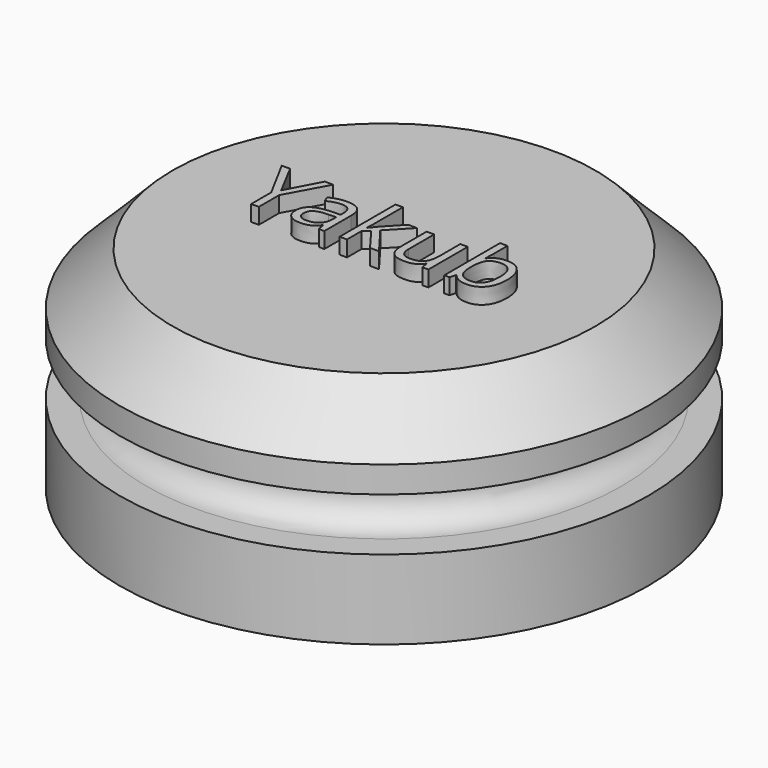
from build123d import *

# Parameters (mm, degrees)
F2_SIZE      = 1
F3_W         = 3.4
F3_H         = 1.1
F4_DEPTH     = 3
F5_R         = 0.49999
F6_TEXT_SIZE = 1.7380913584
F7_DEPTH     = 0.3


# Not quite as in the source:
# - a fillet or chamfer is up to 0.001 mm smaller than in the source, because OpenCascade refuses the exact size
# - Text() gives the source's letters only with a copy of the font that has no kerning and outlines rounded to 1/6400 em; it was checked with that copy


with BuildPart() as f1:
    # F0 (on Front) → F1 (revolve)
    with BuildSketch(Plane.XZ):
        Polygon((5, 4), (0, 4), (0, 0), (5, 0), (5, 1.5), (4, 1.5), (4, 2.5), (5, 2.5), align=None)
    revolve(axis=Axis((0, 0, 2), (0, 0, -1)))

    # F2
    f2_edges = [f1.edges().sort_by_distance(p)[0] for p in [
        (-5, 0, 4),
    ]]
    chamfer(f2_edges, length=F2_SIZE)

    # F3 (on face) → F4 (cut)
    with BuildSketch(Plane(origin=(0, 0, 0), x_dir=(1, 0, 0), z_dir=(0, 0, -1))):
        Rectangle(F3_W, F3_H)
    extrude(amount=-F4_DEPTH, mode=Mode.SUBTRACT)

    # F5 (radius 0.5 in the source; OpenCascade refuses exactly that, so slightly less here)
    f5_edges = [f1.edges().sort_by_distance(p)[0] for p in [
        (-4, 0, 1.5),
        (-4, 0, 2.5),
    ]]
    fillet(f5_edges, radius=F5_R)

    # F6 (on face) → F7 (join)
    with BuildSketch(Plane.XY.offset(4)):
        with Locations((-2.4742341847, -0.5675592284)):
            Text('Yakub', F6_TEXT_SIZE, font='Open Sans', text_align=(TextAlign.LEFT, TextAlign.BOTTOM))
    extrude(amount=F7_DEPTH)


solid = f1.part
